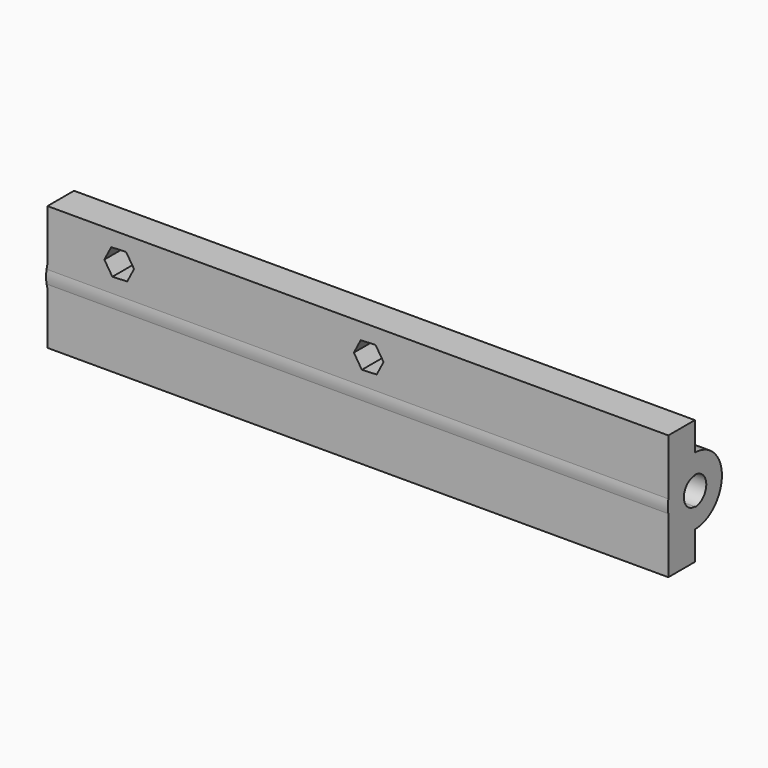
from build123d import *

# Parameters (mm, degrees)
F0_W      = 126.2948513031
F0_H      = 6.7450292408
F1_DEPTH  = 25.4
F4_R      = 2.8033052418
F5_DEPTH  = 127
F6_R      = 6.8744186216
F6_R_2    = 2.9001482236
F7_DEPTH  = 126.492
F9_DEPTH  = 12.7
F11_DEPTH = 12.7


# Not quite as in the source:
# - the program builds the solid bodies; features that only make, move or delete a surface that nothing else refers to are left out


with BuildPart() as f1:
    # F0 (on Top) → F1 (new body)
    with BuildSketch(Plane.XY):
        Rectangle(F0_W, F0_H)
    extrude(amount=F1_DEPTH)

    # F4 (on face) → F5 (cut)
    with BuildSketch(Plane(origin=(-63.1474256516, 0, 0), x_dir=(0, -1, 0), z_dir=(-1, 0, 0))):
        with Locations((-3.3725146204, 12.7)):
            Circle(F4_R)
    extrude(amount=-F5_DEPTH, mode=Mode.SUBTRACT)

    # F6 (on face) → F7 (join)
    with BuildSketch(Plane.YZ.offset(63.1474256516)):
        with Locations((3.3725146204, 12.7)):
            Circle(F6_R)
        with Locations((3.3725146204, 12.7)):
            Circle(F6_R_2, mode=Mode.SUBTRACT)
    extrude(amount=-F7_DEPTH)

    # F8 (on face) → F9 (cut)
    with BuildSketch(Plane.XZ.offset(3.3725146204)):
        Polygon((-45.5430149111, 19.8489452356), (-47.1694619385, 22.3956269569), (-50.1881765182, 22.2604233738), (-51.5804440704, 19.5785380695), (-49.953997043, 17.0318563483), (-46.9352824633, 17.1670599313), align=None)
    extrude(amount=-F9_DEPTH, mode=Mode.SUBTRACT)

    # F10 (on face) → F11 (cut)
    with BuildSketch(Plane.XZ.offset(3.3725146204)):
        Polygon((5.2098441705, 19.6924402974), (3.583397143, 22.2391220187), (0.5646825633, 22.1039184357), (-0.8275849889, 19.4220331314), (0.7988620385, 16.8753514101), (3.8175766182, 17.0105549931), align=None)
    extrude(amount=-F11_DEPTH, mode=Mode.SUBTRACT)


solid = f1.part
